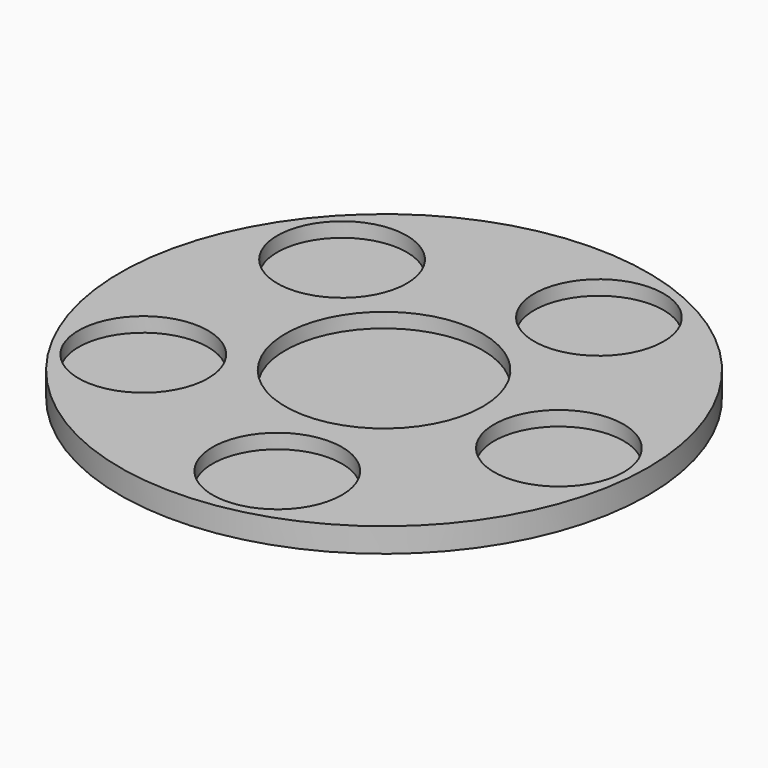
from build123d import *

# Parameters (mm, degrees)
F0_R     = 68.9341581071
F1_DEPTH = 6.35
F2_R     = 25.775239711
F3_DEPTH = 3.81
F5_R     = 16.9134232358
F6_DEPTH = 3.81


# Not quite as in the source:
# - a feature names something its author has since deleted; it is built from what else it names


with BuildPart() as f1:
    # F0 (on Top) → F1 (new body)
    with BuildSketch(Plane.XY):
        Circle(F0_R)
    extrude(amount=F1_DEPTH)

    # F2 (on face) → F3 (cut)
    with BuildSketch(Plane.XY.offset(6.35)):
        Circle(F2_R)
    extrude(amount=-F3_DEPTH, mode=Mode.SUBTRACT)

    # F5 (on face) → F6 (cut)
    with BuildSketch(Plane.XY.offset(6.35)):
        with Locations((-42.6894489161, -25.2584252012)):
            Circle(F5_R)
        with Locations((-37.2139550745, 32.7947959304)):
            Circle(F5_R)
        with Locations((19.6899598242, 45.5267237403)):
            Circle(F5_R)
        with Locations((49.383019483, -4.6577332624)):
            Circle(F5_R)
        with Locations((10.8304246834, -48.405361207)):
            Circle(F5_R)
    extrude(amount=-F6_DEPTH, mode=Mode.SUBTRACT)


solid = f1.part
